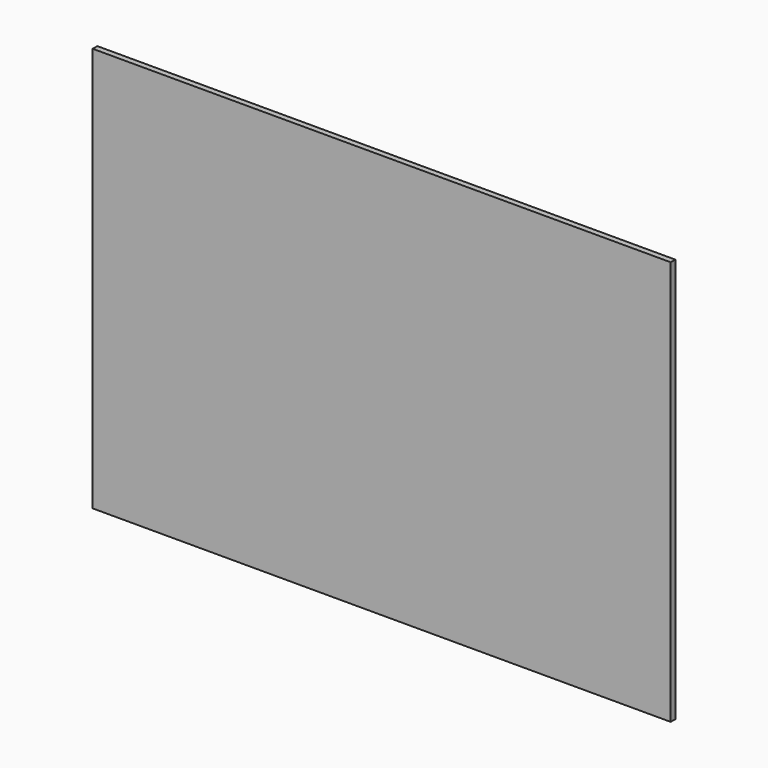
from build123d import *

# Parameters (mm, degrees)
F0_W     = 254
F0_H     = 177.8
F1_DEPTH = 2.54


# Not quite as in the source:
# - a feature names something its author has since deleted; it is built from what else it names


with BuildPart() as f1:
    # F0 (on Front) → F1 (new body)
    with BuildSketch(Plane.XZ):
        with Locations((5.9266667813, -47.5251817665)):
            Rectangle(F0_W, F0_H)
    extrude(amount=F1_DEPTH)


solid = f1.part
